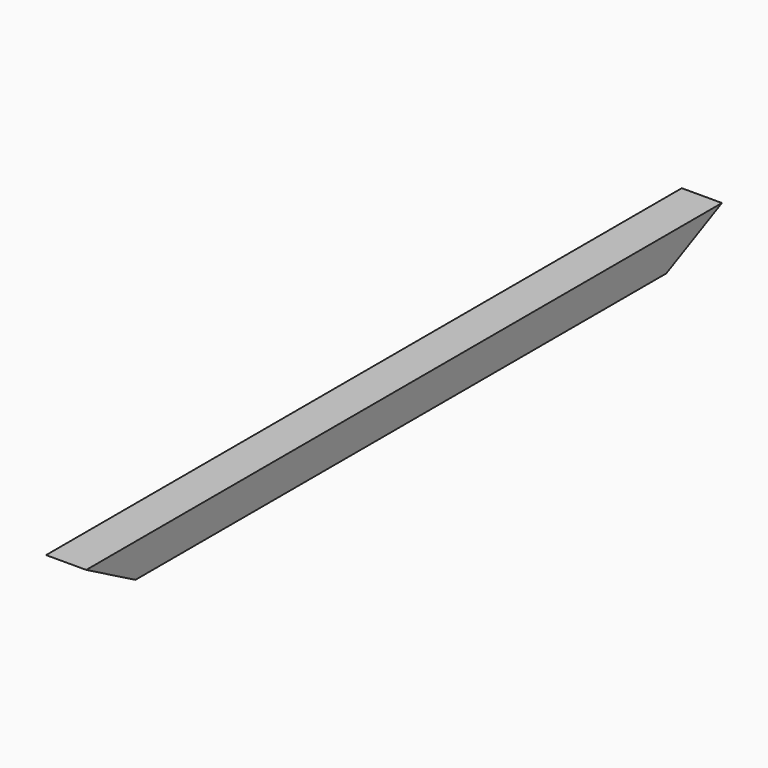
from build123d import *

# Parameters (mm, degrees)
F1_DEPTH      = 2540
F3_DEPTH      = 127.001
F3_DEPTH_BACK = 127.001


# Not quite as in the source:
# - a pattern or mirror of a feature is missing from the dataset's text; its kind, count and spacing are read off the source's solid


with BuildPart() as f1:
    # F0 (on Front) → F1 (new body, symmetric)
    with BuildSketch(Plane.XZ):
        with BuildLine():
            Line((-127, 0), (-106.8393477338, -230.4373098607))
            ThreePointArc((-106.8393477338, -230.4373098607), (0, -254), (106.8393477338, -230.4373098607))
            Line((106.8393477338, -230.4373098607), (127, 0))
            Line((127, 0), (-127, 0))
        make_face()
    extrude(amount=F1_DEPTH, both=True)

    # F2 (on Right) → F3 (cut, two sides)
    with BuildSketch(Plane.YZ) as f3_sk:
        Polygon((-1970.9674119949, -301.9396364689), (-2584.4640731812, 39.0566559158), (-2584.4640731812, -301.9396364689), align=None)
    f3 = extrude(amount=F3_DEPTH, mode=Mode.SUBTRACT) + extrude(f3_sk.sketch, amount=-F3_DEPTH_BACK, mode=Mode.SUBTRACT)

    # F3_copies: F3 across plane
    add(f3.mirror(Plane.ZX), mode=Mode.SUBTRACT)


solid = f1.part
